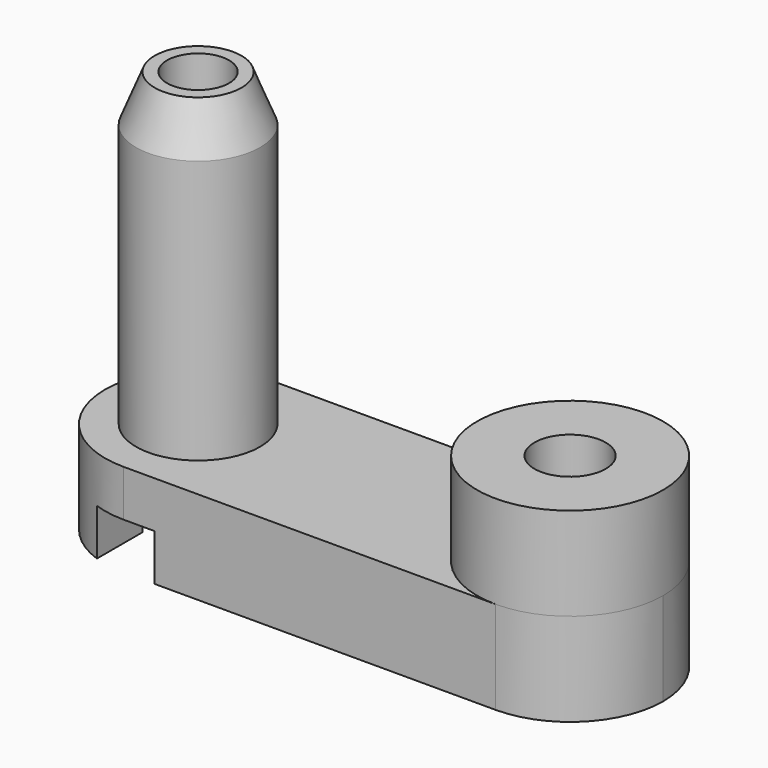
from build123d import *

# Parameters (mm, degrees)
F0_W      = 18
F0_H      = 6
F1_DEPTH  = 3
F2_R      = 3
F2_R_2    = 2
F3_DEPTH  = 10
F4_R      = 1
F4_R_2    = 1.15
F5_DEPTH  = 20
F6_SIZE2  = 1.5
F6_SIZE   = 0.6
F7_W      = 11.6012076614
F7_H      = 11.8295210414
F8_DEPTH  = 7
F9_R      = 2.9999
F10_W     = 5.4413094251
F10_H     = 2
F11_DEPTH = 1.5


# Not quite as in the source:
# - a fillet or chamfer is up to 0.001 mm smaller than in the source, because OpenCascade refuses the exact size


with BuildPart() as f1:
    # F0 (on Top) → F1 (new body)
    with BuildSketch(Plane.XY):
        with Locations((1.8924829921, 0)):
            Rectangle(F0_W, F0_H)
    extrude(amount=F1_DEPTH)

    # F2 (on face) → F3 (join)
    with BuildSketch(Plane.XY.offset(3)):
        with Locations((7.8924829921, 0)):
            Circle(F2_R)
        with Locations((-4.1075170079, 0)):
            Circle(F2_R_2)
    extrude(amount=F3_DEPTH)

    # F4 (on face) → F5 (cut)
    with BuildSketch(Plane.XY.offset(13)):
        with Locations((-4.1075170079, 0)):
            Circle(F4_R)
        with Locations((7.8924829921, 0)):
            Circle(F4_R_2)
    extrude(amount=-F5_DEPTH, mode=Mode.SUBTRACT)

    # F6
    f6_edges = [f1.edges().sort_by_distance(p)[0] for p in [
        (-6.107517, 0, 13),
    ]]
    f6_side = f1.faces().sort_by_distance((-6.050948, 0, 13))[0]
    chamfer(f6_edges, length=F6_SIZE, length2=F6_SIZE2, reference=f6_side)

    # F7 (on face) → F8 (cut)
    with BuildSketch(Plane.XY.offset(13)):
        with Locations((7.5882198871, -0.5373002496)):
            Rectangle(F7_W, F7_H)
    extrude(amount=-F8_DEPTH, mode=Mode.SUBTRACT)

    # F9 (radius 3 in the source; OpenCascade refuses exactly that, so slightly less here)
    f9_edges = [f1.edges().sort_by_distance(p)[0] for p in [
        (10.892483, -3, 1.5),
        (10.892483, 3, 1.5),
        (-7.107517, 3, 1.5),
        (-7.107517, -3, 1.5),
    ]]
    fillet(f9_edges, radius=F9_R)

    # F10 (on face) → F11 (cut)
    with BuildSketch(Plane(origin=(0, 0, 0), x_dir=(1, 0, 0), z_dir=(0, 0, -1))):
        Polygon((-3.1075170079, 5.622364855), (-5.1075170079, 5.622364855), (-5.1075170079, 1), (-5.1075170079, -1), (-5.1075170079, -5.5661949279), (-3.1075170079, -5.5661949279), align=None)
        with Locations((-7.8281717205, 0)):
            Rectangle(F10_W, F10_H)
    extrude(amount=-F11_DEPTH, mode=Mode.SUBTRACT)


solid = f1.part
